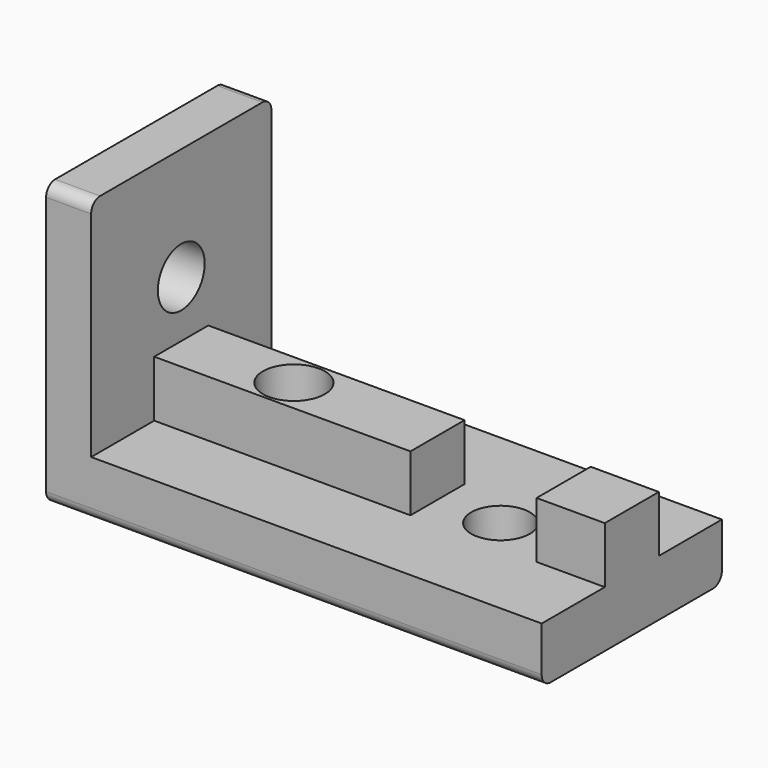
from build123d import *

# Parameters (mm, degrees)
F0_W      = 40
F0_H      = 20
F1_DEPTH  = 5
F2_W      = 40
F2_H      = 6
F3_DEPTH  = 5
F4_R      = 2.75
F5_DEPTH  = 25
F6_W      = 11.2
F6_H      = 6
F7_DEPTH  = 5
F8_R      = 2.6
F9_DEPTH  = 5
F10_R     = 2.6
F11_DEPTH = 4
F12_R     = 1


# Not quite as in the source:
# - a fillet or chamfer that OpenCascade refuses, or shapes differently, is made with other operations: its cross-section is extruded or revolved along the edge and cut away or added
# - a feature names something its author has since deleted; it is built from what else it names


with BuildPart() as f1:
    # F0 (on Top) → F1 (new body)
    with BuildSketch(Plane.XY):
        with Locations((20, 0)):
            Rectangle(F0_W, F0_H)
    extrude(amount=F1_DEPTH)

    # F2 (on face) → F3 (join)
    with BuildSketch(Plane.XY.offset(5)):
        with Locations((20, 0)):
            Rectangle(F2_W, F2_H)
    extrude(amount=F3_DEPTH)

    # F4 (on face) → F5 (cut)
    with BuildSketch(Plane.XY.offset(10)):
        with Locations((10, 0)):
            Circle(F4_R)
    extrude(amount=-F5_DEPTH, mode=Mode.SUBTRACT)

    # F6 (on face) → F7 (cut, through all)
    with BuildSketch(Plane.XY.offset(10)):
        with Locations((28.35, 0)):
            Rectangle(F6_W, F6_H)
    extrude(amount=-F7_DEPTH, mode=Mode.SUBTRACT)

    # F8 (on face) → F9 (cut, through all)
    with BuildSketch(Plane.XY.offset(5)):
        with Locations((28.35, 0)):
            Circle(F8_R)
    extrude(amount=-F9_DEPTH, mode=Mode.SUBTRACT)

    # F10 (on face) → F11 (join)
    with BuildSketch(Plane(origin=(0, 0, 0), x_dir=(0, -1, 0), z_dir=(-1, 0, 0))):
        Polygon((-10, 25), (-10, 5), (-3, 5), (-3, 10), (3, 10), (3, 5), (10, 5), (10, 25), align=None)
        with Locations((0, 15)):
            Circle(F10_R, mode=Mode.SUBTRACT)
        Polygon((-10, 5), (-10, 0), (10, 0), (10, 5), (3, 5), (3, 10), (-3, 10), (-3, 5), align=None)
    extrude(amount=F11_DEPTH)

    # F12
    f12_edges = [f1.edges().sort_by_distance(p)[0] for p in [
        (-2, -10, 25),
        (-2, 10, 25),
        (18, -10, 0),
        (18, 10, 0),
    ]]
    fillet(f12_edges, radius=F12_R)

    # F13: chamfer of 0.5 x 0.2886751346 on 1 edges, made by hand

    # F13_s1 → F13_t2 (revolve, cut)
    with BuildSketch(Plane.XZ):
        Polygon((13.0386751346, 0), (12.75, 0.5), (12.75, 0), align=None)
    revolve(axis=Axis((10, 0, 0), (0, 0, 1)), mode=Mode.SUBTRACT)


solid = f1.part
